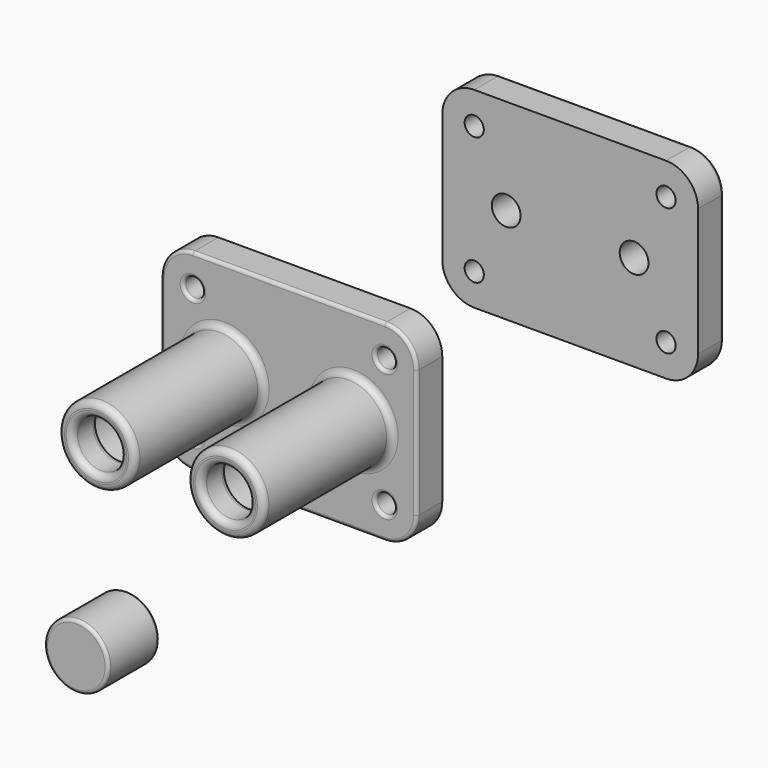
from build123d import *

# Parameters (mm, degrees)
F1_DEPTH  = 5
F2_D      = 4.5
F3_D      = 3
F4_R      = 0.5
F7_R      = 6
F7_R_2    = 4.5
F8_DEPTH  = 25
F9_R      = 6
F9_R_2    = 4.5
F9_R_3    = 3.75
F10_DEPTH = 5
F13_R     = 5
F14_DEPTH = 10
F15_D     = 4.5
F15_DEPTH = 7
F15_TIP   = 1.3519363928
F16_R     = 0.5


# Not quite as in the source:
# - a fillet or chamfer that OpenCascade refuses, or shapes differently, is made with other operations: its cross-section is extruded or revolved along the edge and cut away or added


with BuildPart() as f1:
    # F0 (on Front) → F1 (new body)
    with BuildSketch(Plane.XZ):
        with BuildLine():
            Line((15, 15), (-15, 15))
            ThreePointArc((-15, 15), (-18.5355339059, 13.5355339059), (-20, 10))
            Line((-20, 10), (-20, -10))
            ThreePointArc((-20, -10), (-18.5355339059, -13.5355339059), (-15, -15))
            Line((-15, -15), (15, -15))
            ThreePointArc((15, -15), (18.5355339059, -13.5355339059), (20, -10))
            Line((20, -10), (20, 10))
            ThreePointArc((20, 10), (18.5355339059, 13.5355339059), (15, 15))
        make_face()
    extrude(amount=-F1_DEPTH)

    # F2 (through all)
    with Locations(Plane.XZ):
        with Locations((-10, 0), (10, 0)):
            Hole(F2_D / 2)

    # F3 (through all)
    with Locations(Plane.XZ):
        with Locations((-15, 10), (15, 10), (15, -10), (-15, -10)):
            Hole(F3_D / 2)

    # F4
    f4_edges = [f1.edges().sort_by_distance(p)[0] for p in [
        (0, 0, 15),
        (-18.535534, 0, 13.535534),
        (18.535534, 0, 13.535534),
        (20, 0, 0),
        (-20, 0, 0),
        (18.535534, 0, -13.535534),
        (-18.535534, 0, -13.535534),
        (0, 0, -15),
        (-16.5, 0, -10),
        (13.5, 0, -10),
        (-12.25, 0, 0),
        (-16.5, 0, 10),
        (7.75, 0, 0),
        (13.5, 0, 10),
    ]]
    fillet(f4_edges, radius=F4_R)


with BuildPart() as f6_1:
    # F6: instance of F1
    add(f1.part.mirror(Plane(origin=(0, 30, 0), x_dir=(1, 0, 0), z_dir=(0, 1, 0))))


with BuildPart() as f1_1:
    add(f1.part)

    # F7 (on face) → F8 (join)
    with BuildSketch(Plane.XZ):
        with Locations((10.0867114961, 0)):
            Circle(F7_R)
        with Locations((10.0867114961, 0)):
            Circle(F7_R_2, mode=Mode.SUBTRACT)
        with Locations((-10.0867114961, 0)):
            Circle(F7_R)
        with Locations((-10.0867114961, 0)):
            Circle(F7_R_2, mode=Mode.SUBTRACT)
    extrude(amount=F8_DEPTH)

    # F9 (on face) → F10 (join)
    with BuildSketch(Plane.XZ.offset(25)):
        with Locations((10.0867114961, 0)):
            Circle(F9_R)
        with Locations((10.0867114961, 0)):
            Circle(F9_R_2, mode=Mode.SUBTRACT)
        with Locations((-10.0867114961, 0)):
            Circle(F9_R)
        with Locations((-10.0867114961, 0)):
            Circle(F9_R_3, mode=Mode.SUBTRACT)
        with Locations((10.0867114961, 0)):
            Circle(F9_R_2)
        with Locations((10.0867114961, 0)):
            Circle(F9_R_3, mode=Mode.SUBTRACT)
    extrude(amount=-F10_DEPTH)

    # F11: fillet of radius 1 on 8 edges, made by hand

    # F11_s1 → F11_t2 (revolve)
    with BuildSketch(Plane.XY):
        with BuildLine():
            ThreePointArc((-3.0867114961, 0), (-3.7938182773, -0.2928932188), (-4.0867114961, -1))
            Line((-4.0867114961, -1), (-4.0867114961, 0))
            Line((-4.0867114961, 0), (-3.0867114961, 0))
        make_face()
    revolve(axis=Axis((-10.0867114961, 0, 0), (0, -1, 0)))

    # F11_s3 → F11_t4 (revolve)
    with BuildSketch(Plane.XY):
        with BuildLine():
            ThreePointArc((17.0867114961, 0), (16.3796047149, -0.2928932188), (16.0867114961, -1))
            Line((16.0867114961, -1), (16.0867114961, 0))
            Line((16.0867114961, 0), (17.0867114961, 0))
        make_face()
    revolve(axis=Axis((10.0867114961, 0, 0), (0, -1, 0)))

    # F11_s5 → F11_t6 (revolve, cut)
    with BuildSketch(Plane.XY):
        with BuildLine():
            ThreePointArc((16.0867114961, -24), (15.7938182773, -24.7071067812), (15.0867114961, -25))
            Line((15.0867114961, -25), (16.0867114961, -25))
            Line((16.0867114961, -25), (16.0867114961, -24))
        make_face()
    revolve(axis=Axis((10.0867114961, -25, 0), (0, -1, 0)), mode=Mode.SUBTRACT)

    # F11_s7 → F11_t8 (revolve, cut)
    with BuildSketch(Plane.XY):
        with BuildLine():
            ThreePointArc((14.8367114961, -25), (14.1296047149, -24.7071067812), (13.8367114961, -24))
            Line((13.8367114961, -24), (13.8367114961, -25))
            Line((13.8367114961, -25), (14.8367114961, -25))
        make_face()
    revolve(axis=Axis((10.0867114961, -25, 0), (0, -1, 0)), mode=Mode.SUBTRACT)

    # F11_s9 → F11_t10 (revolve, cut)
    with BuildSketch(Plane.XY):
        with BuildLine():
            ThreePointArc((14.5867114961, -20), (14.0461420811, -20.3558734009), (13.8367114961, -20.9682458366))
            Line((13.8367114961, -20.9682458366), (13.8367114961, -20))
            Line((13.8367114961, -20), (14.5867114961, -20))
        make_face()
    revolve(axis=Axis((10.0867114961, -20, 0), (0, -1, 0)), mode=Mode.SUBTRACT)

    # F11_s11 → F11_t12 (revolve, cut)
    with BuildSketch(Plane.XY):
        with BuildLine():
            ThreePointArc((-4.0867114961, -24), (-4.3796047149, -24.7071067812), (-5.0867114961, -25))
            Line((-5.0867114961, -25), (-4.0867114961, -25))
            Line((-4.0867114961, -25), (-4.0867114961, -24))
        make_face()
    revolve(axis=Axis((-10.0867114961, -25, 0), (0, -1, 0)), mode=Mode.SUBTRACT)

    # F11_s13 → F11_t14 (revolve, cut)
    with BuildSketch(Plane.XY):
        with BuildLine():
            ThreePointArc((-5.3367114961, -25), (-6.0438182773, -24.7071067812), (-6.3367114961, -24))
            Line((-6.3367114961, -24), (-6.3367114961, -25))
            Line((-6.3367114961, -25), (-5.3367114961, -25))
        make_face()
    revolve(axis=Axis((-10.0867114961, -25, 0), (0, -1, 0)), mode=Mode.SUBTRACT)

    # F11_s15 → F11_t16 (revolve, cut)
    with BuildSketch(Plane.XY):
        with BuildLine():
            ThreePointArc((-5.5867114961, -20), (-6.1272809112, -20.3558734009), (-6.3367114961, -20.9682458366))
            Line((-6.3367114961, -20.9682458366), (-6.3367114961, -20))
            Line((-6.3367114961, -20), (-5.5867114961, -20))
        make_face()
    revolve(axis=Axis((-10.0867114961, -20, 0), (0, -1, 0)), mode=Mode.SUBTRACT)


with BuildPart() as f14:
    # F13 (on offset) → F14 (new body)
    with BuildSketch(Plane.XZ.offset(50)):
        with Locations((14.7593151778, -6.616268307)):
            Circle(F13_R)
    extrude(amount=F14_DEPTH)

    # F15
    with Locations(Plane(origin=(0, -50, 0), x_dir=(1, 0, 0), z_dir=(0, 1, 0))):
        with Locations((14.7593151778, 6.616268307)):
            Hole(F15_D / 2, depth=F15_DEPTH)
            with Locations((0, 0, -(F15_DEPTH + F15_TIP / 2))):  # 118° drill point
                Cone(0, F15_D / 2, F15_TIP, mode=Mode.SUBTRACT)

    # F16
    f16_edges = [f14.edges().sort_by_distance(p)[0] for p in [
        (9.759315, -60, -6.616268),
        (9.759315, -50, -6.616268),
    ]]
    fillet(f16_edges, radius=F16_R)


solid = Compound([f6_1.part, f1_1.part, f14.part])
